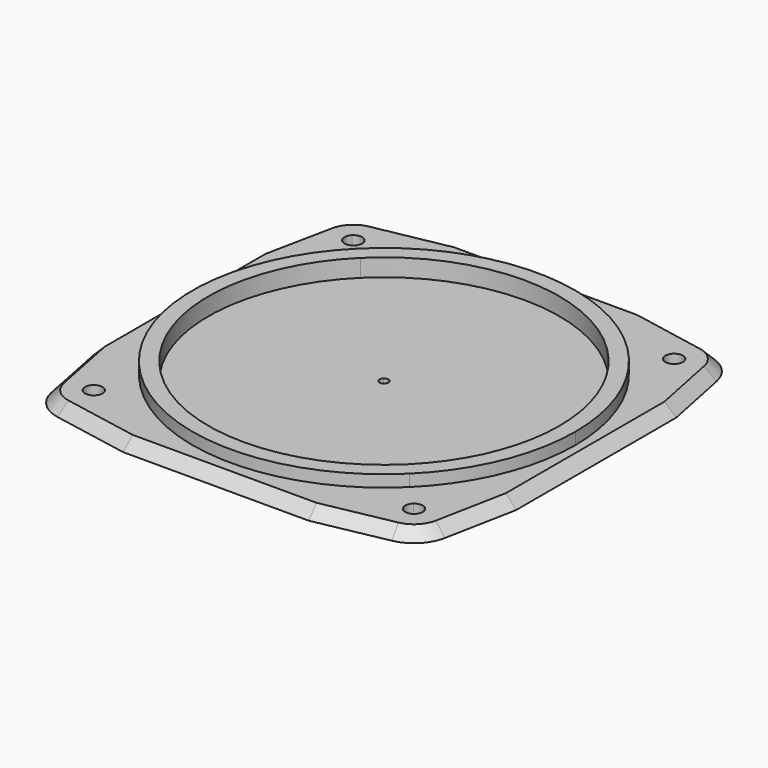
from build123d import *

# Parameters (mm, degrees)
F1_DEPTH     = 0.762
F2_DEPTH     = 3.302
F3_DEPTH     = 1.5875
F4_T1_DEPTH  = 68.7698589568
F4_T3_DEPTH  = 29.8890950425
F4_T5_DEPTH  = 30.9975051116
F4_T7_DEPTH  = 66.2764134385
F4_T9_DEPTH  = 29.6095967996
F4_T11_DEPTH = 30.7124717043
F4_T13_DEPTH = 66.1433332478
F4_T15_DEPTH = 30.7409380137
F4_T17_DEPTH = 29.6692094887
F4_T19_DEPTH = 68.3706865963
F4_T21_DEPTH = 30.237608237
F4_T23_DEPTH = 30.2773753002
F4_T26_ANGLE = 67.887600788
F4_T28_ANGLE = 67.7694142572
F4_T30_ANGLE = 67.6911456036
F4_T32_ANGLE = 68.1706761996


# Not quite as in the source:
# - a fillet or chamfer that OpenCascade refuses, or shapes differently, is made with other operations: its cross-section is extruded or revolved along the edge and cut away or added


with BuildPart() as f1:
    # F0 (on Top) → F1 (new body)
    with BuildSketch(Plane.XY):
        with BuildLine():
            Line((0.4463481019, 0.4516617893), (17.8539240764, 18.0664715723))
            ThreePointArc((17.8539240764, 18.0664715723), (0, 25.4), (-17.8539240764, 18.0664715723))
            Line((-17.8539240764, 18.0664715723), (-0.4463481019, 0.4516617893))
            ThreePointArc((-0.4463481019, 0.4516617893), (0, 0.635), (0.4463481019, 0.4516617893))
        make_face()
        with BuildLine():
            Line((-0.4463481019, 0.4516617893), (-17.8539240764, 18.0664715723))
            ThreePointArc((-17.8539240764, 18.0664715723), (-25.4, 0), (-17.8539240764, -18.0664715723))
            Line((-17.8539240764, -18.0664715723), (-0.4463481019, -0.4516617893))
            ThreePointArc((-0.4463481019, -0.4516617893), (-0.635, 0), (-0.4463481019, 0.4516617893))
        make_face()
        with BuildLine():
            ThreePointArc((-17.8539240764, -18.0664715723), (0, -25.4), (17.8539240764, -18.0664715723))
            Line((17.8539240764, -18.0664715723), (0.4463481019, -0.4516617893))
            ThreePointArc((0.4463481019, -0.4516617893), (0, -0.635), (-0.4463481019, -0.4516617893))
            Line((-0.4463481019, -0.4516617893), (-17.8539240764, -18.0664715723))
        make_face()
        with BuildLine():
            ThreePointArc((17.8539240764, -18.0664715723), (23.4376798291, -9.789543617), (25.4, 0))
            ThreePointArc((25.4, 0), (23.4376798291, 9.789543617), (17.8539240764, 18.0664715723))
            Line((17.8539240764, 18.0664715723), (0.4463481019, 0.4516617893))
            ThreePointArc((0.4463481019, 0.4516617893), (0.5859419957, 0.2447385904), (0.635, 0))
            ThreePointArc((0.635, 0), (0.5859419957, -0.2447385904), (0.4463481019, -0.4516617893))
            Line((0.4463481019, -0.4516617893), (17.8539240764, -18.0664715723))
        make_face()
    extrude(amount=F1_DEPTH)

    # F0 (on Top) → F2 (join)
    with BuildSketch(Plane.XY):
        with BuildLine():
            ThreePointArc((-17.8539240764, 18.0664715723), (0, 25.4), (17.8539240764, 18.0664715723))
            Line((17.8539240764, 18.0664715723), (19.4706182402, 19.7024121658))
            ThreePointArc((19.4706182402, 19.7024121658), (0, 27.7000003576), (-19.4706182402, 19.7024121658))
            Line((-19.4706182402, 19.7024121658), (-17.8539240764, 18.0664715723))
        make_face()
        with BuildLine():
            ThreePointArc((-17.8539240764, -18.0664715723), (-25.4, 0), (-17.8539240764, 18.0664715723))
            Line((-17.8539240764, 18.0664715723), (-19.4706182402, 19.7024121658))
            ThreePointArc((-19.4706182402, 19.7024121658), (-27.7000003576, 0), (-19.4706182402, -19.7024121658))
            Line((-19.4706182402, -19.7024121658), (-17.8539240764, -18.0664715723))
        make_face()
        with BuildLine():
            Line((19.4706182402, -19.7024121658), (17.8539240764, -18.0664715723))
            ThreePointArc((17.8539240764, -18.0664715723), (0, -25.4), (-17.8539240764, -18.0664715723))
            Line((-17.8539240764, -18.0664715723), (-19.4706182402, -19.7024121658))
            ThreePointArc((-19.4706182402, -19.7024121658), (0, -27.7000003576), (19.4706182402, -19.7024121658))
        make_face()
        with BuildLine():
            ThreePointArc((17.8539240764, 18.0664715723), (23.4376798291, 9.789543617), (25.4, 0))
            ThreePointArc((25.4, 0), (23.4376798291, -9.789543617), (17.8539240764, -18.0664715723))
            Line((17.8539240764, -18.0664715723), (19.4706182402, -19.7024121658))
            ThreePointArc((19.4706182402, -19.7024121658), (25.5599897498, -10.6759984918), (27.7000003576, 0))
            ThreePointArc((27.7000003576, 0), (25.5599897498, 10.6759984918), (19.4706182402, 19.7024121658))
            Line((19.4706182402, 19.7024121658), (17.8539240764, 18.0664715723))
        make_face()
    extrude(amount=F2_DEPTH)

    # F0 (on Top) → F3 (join)
    with BuildSketch(Plane.XY):
        with BuildLine():
            ThreePointArc((-19.4706182402, 19.7024121658), (0, 27.7000003576), (19.4706182402, 19.7024121658))
            Line((19.4706182402, 19.7024121658), (22.3259415659, 22.5917275607))
            ThreePointArc((22.3259415659, 22.5917275607), (22.3153141911, 24.3877473432), (24.1113339735, 24.398374718))
            Line((24.1113339735, 24.398374718), (26.7918864226, 27.1108386229))
            Line((26.7918864226, 27.1108386229), (27.6821187888, 28.0116690324))
            ThreePointArc((27.6821187888, 28.0116690324), (26.1722118102, 29.1163410613), (24.4059253481, 29.7330675073))
            Line((24.4059253481, 29.7330675073), (13.4577511535, 31.8168438971))
            Line((13.4577511535, 31.8168438971), (-13.4931333577, 31.8168438971))
            Line((-13.4931333577, 31.8168438971), (-24.4124478948, 29.7336912681))
            ThreePointArc((-24.4124478948, 29.7336912681), (-26.1764044214, 29.1172901956), (-27.6845826781, 28.0141622538))
            Line((-27.6845826781, 28.0141622538), (-26.7918864226, 27.1108386229))
            Line((-26.7918864226, 27.1108386229), (-24.1137970362, 24.4008671029))
            ThreePointArc((-24.1137970362, 24.4008671029), (-22.7321077122, 24.6676976509), (-21.952476244, 23.4961863607))
            ThreePointArc((-21.952476244, 23.4961863607), (-22.0502202295, 23.007600814), (-22.328406695, 22.5942220368))
            Line((-22.328406695, 22.5942220368), (-19.4706182402, 19.7024121658))
        make_face()
        with BuildLine():
            ThreePointArc((-19.4706182402, -19.7024121658), (-27.7000003576, 0), (-19.4706182402, 19.7024121658))
            Line((-19.4706182402, 19.7024121658), (-22.328406695, 22.5942220368))
            ThreePointArc((-22.328406695, 22.5942220368), (-24.1257998226, 22.6034901569), (-24.1137970362, 24.4008671029))
            Line((-24.1137970362, 24.4008671029), (-26.7918864226, 27.1108386229))
            Line((-26.7918864226, 27.1108386229), (-27.6845826781, 28.0141622538))
            ThreePointArc((-27.6845826781, 28.0141622538), (-28.806546627, 26.5195384668), (-29.4448227731, 24.7630342884))
            Line((-29.4448227731, 24.7630342884), (-31.4425267279, 14.9509597699))
            Line((-31.4425267279, 14.9509597699), (-31.4425267279, -14.6264504503))
            Line((-31.4425267279, -14.6264504503), (-29.4338375739, -24.7214172456))
            ThreePointArc((-29.4338375739, -24.7214172456), (-28.7971534061, -26.4922974633), (-27.669411804, -27.9988107734))
            Line((-27.669411804, -27.9988107734), (-26.7918864226, -27.1108386229))
            Line((-26.7918864226, -27.1108386229), (-24.0986269887, -24.385516459))
            ThreePointArc((-24.0986269887, -24.385516459), (-24.1092543635, -22.5894966765), (-22.3132345811, -22.5788693018))
            Line((-22.3132345811, -22.5788693018), (-19.4706182402, -19.7024121658))
        make_face()
        with BuildLine():
            Line((22.3230898006, -22.5888418457), (19.4706182402, -19.7024121658))
            ThreePointArc((19.4706182402, -19.7024121658), (0, -27.7000003576), (-19.4706182402, -19.7024121658))
            Line((-19.4706182402, -19.7024121658), (-22.3132345811, -22.5788693018))
            ThreePointArc((-22.3132345811, -22.5788693018), (-22.0340467935, -22.9927156995), (-21.9359307849, -23.4821928804))
            ThreePointArc((-21.9359307849, -23.4821928804), (-22.7164536041, -24.6540768718), (-24.0986269887, -24.385516459))
            Line((-24.0986269887, -24.385516459), (-26.7918864226, -27.1108386229))
            Line((-26.7918864226, -27.1108386229), (-27.669411804, -27.9988107734))
            ThreePointArc((-27.669411804, -27.9988107734), (-26.1496583495, -29.1086454062), (-24.3713676477, -29.724328486))
            Line((-24.3713676477, -29.724328486), (-13.163754974, -31.8168438971))
            Line((-13.163754974, -31.8168438971), (13.9202097279, -31.8168438971))
            Line((13.9202097279, -31.8168438971), (24.4012740355, -29.7591081974))
            ThreePointArc((24.4012740355, -29.7591081974), (26.1707747188, -29.1285461533), (27.6783635387, -28.0078690768))
            Line((27.6783635387, -28.0078690768), (26.7918864226, -27.1108386229))
            Line((26.7918864226, -27.1108386229), (24.1069762986, -24.3939651657))
            ThreePointArc((24.1069762986, -24.3939651657), (22.2746158391, -24.4207569441), (22.3230898006, -22.5888418457))
        make_face()
        with BuildLine():
            Line((22.3259415659, 22.5917275607), (19.4706182402, 19.7024121658))
            ThreePointArc((19.4706182402, 19.7024121658), (25.5599897498, 10.6759984918), (27.7000003576, 0))
            ThreePointArc((27.7000003576, 0), (25.5599897498, -10.6759984918), (19.4706182402, -19.7024121658))
            Line((19.4706182402, -19.7024121658), (22.3230898006, -22.5888418457))
            ThreePointArc((22.3230898006, -22.5888418457), (23.6913792809, -22.3664758287), (24.4479394177, -23.5280607403))
            ThreePointArc((24.4479394177, -23.5280607403), (24.3596282174, -23.9933687895), (24.1069762986, -24.3939651657))
            Line((24.1069762986, -24.3939651657), (26.7918864226, -27.1108386229))
            Line((26.7918864226, -27.1108386229), (27.6783635387, -28.0078690768))
            ThreePointArc((27.6783635387, -28.0078690768), (28.7879487003, -26.5030054203), (29.411169277, -24.7402263734))
            Line((29.411169277, -24.7402263734), (31.4425267279, -14.2945268971))
            Line((31.4425267279, -14.2945268971), (31.4425267279, 14.8837109626))
            Line((31.4425267279, 14.8837109626), (29.4421670292, 24.7560759433))
            ThreePointArc((29.4421670292, 24.7560759433), (28.8045816259, 26.5149404148), (27.6821187888, 28.0116690324))
            Line((27.6821187888, 28.0116690324), (26.7918864226, 27.1108386229))
            Line((26.7918864226, 27.1108386229), (24.1113339735, 24.398374718))
            ThreePointArc((24.1113339735, 24.398374718), (24.3905217612, 23.9845283202), (24.4886377697, 23.4950511393))
            ThreePointArc((24.4886377697, 23.4950511393), (23.7081149506, 22.3231671479), (22.3259415659, 22.5917275607))
        make_face()
    extrude(amount=F3_DEPTH)

    # F4: chamfer of 2.54 on 12 edges, made by hand

    # F4_s2 → F4_t1 (cut)
    with BuildSketch(Plane.XZ.offset(-34.5471841382)):
        Polygon((-28.9025267279, 1.5875), (-31.4425267279, -0.9525), (-31.4425267279, 1.5875), align=None)
    extrude(amount=F4_T1_DEPTH, mode=Mode.SUBTRACT)

    # F4_s4 → F4_t3 (cut)
    with BuildSketch(Plane(origin=(-2.2222353061, 11.168174818, 0), x_dir=(0, 0, 1), z_dir=(0.1951534433, -0.9807727227, 0))):
        Polygon((1.5875, 31.1523747161), (-0.9525, 33.6923747161), (1.5875, 33.6923747161), align=None)
    extrude(amount=F4_T3_DEPTH, mode=Mode.SUBTRACT)

    # F4_s6 → F4_t5 (cut)
    with BuildSketch(Plane(origin=(-18.1876927678, 3.3957300736, 0), x_dir=(0, 0, 1), z_dir=(0.9830134812, -0.1835333642, 0))):
        Polygon((1.5875, 31.1523747161), (-0.9525, 33.6923747161), (1.5875, 33.6923747161), align=None)
    extrude(amount=F4_T5_DEPTH, mode=Mode.SUBTRACT)

    # F4_s8 → F4_t7 (cut)
    with BuildSketch(Plane.YZ.offset(-32.7599793423)):
        Polygon((-29.2768438971, 1.5875), (-31.8168438971, -0.9525), (-31.8168438971, 1.5875), align=None)
    extrude(amount=F4_T7_DEPTH, mode=Mode.SUBTRACT)

    # F4_s10 → F4_t9 (cut)
    with BuildSketch(Plane(origin=(3.6690463267, 18.0211666908, 0), x_dir=(0, 0, 1), z_dir=(-0.1995036107, -0.9798970912, 0))):
        Polygon((1.5875, 31.2532109374), (-0.9525, 33.7932109374), (1.5875, 33.7932109374), align=None)
    extrude(amount=F4_T9_DEPTH, mode=Mode.SUBTRACT)

    # F4_s12 → F4_t11 (cut)
    with BuildSketch(Plane(origin=(12.0865328675, 2.3058308864, 0), x_dir=(0, 0, 1), z_dir=(-0.9822842374, -0.1873971104, 0))):
        Polygon((1.5875, 31.2417584447), (-0.9525, 33.7817584447), (1.5875, 33.7817584447), align=None)
    extrude(amount=F4_T11_DEPTH, mode=Mode.SUBTRACT)

    # F4_s14 → F4_t13 (cut)
    with BuildSketch(Plane.YZ.offset(-33.089357726)):
        Polygon((29.2768438971, 1.5875), (31.8168438971, -0.9525), (31.8168438971, 1.5875), align=None)
    extrude(amount=F4_T13_DEPTH, mode=Mode.SUBTRACT)

    # F4_s16 → F4_t15 (cut)
    with BuildSketch(Plane(origin=(18.0914247696, -3.4433580544, 0), x_dir=(0, 0, 1), z_dir=(-0.9823647823, 0.1869744218, 0))):
        Polygon((1.5875, 31.2320021705), (-0.9525, 33.7720021705), (1.5875, 33.7720021705), align=None)
    extrude(amount=F4_T15_DEPTH, mode=Mode.SUBTRACT)

    # F4_s18 → F4_t17 (cut)
    with BuildSketch(Plane(origin=(2.2346970165, -11.0288887457, 0), x_dir=(0, 0, 1), z_dir=(-0.1985865833, 0.980083348, 0))):
        Polygon((1.5875, 31.2320021705), (-0.9525, 33.7720021705), (1.5875, 33.7720021705), align=None)
    extrude(amount=F4_T17_DEPTH, mode=Mode.SUBTRACT)

    # F4_s20 → F4_t19 (cut)
    with BuildSketch(Plane.XZ.offset(-34.4799353309)):
        Polygon((28.9025267279, 1.5875), (31.4425267279, -0.9525), (31.4425267279, 1.5875), align=None)
    extrude(amount=F4_T19_DEPTH, mode=Mode.SUBTRACT)

    # F4_s22 → F4_t21 (cut)
    with BuildSketch(Plane(origin=(-3.5641324861, -18.3275753981, 0), x_dir=(0, 0, 1), z_dir=(0.1908922257, 0.9816110015, 0))):
        Polygon((1.5875, 31.053044204), (-0.9525, 33.593044204), (1.5875, 33.593044204), align=None)
    extrude(amount=F4_T21_DEPTH, mode=Mode.SUBTRACT)

    # F4_s24 → F4_t23 (cut)
    with BuildSketch(Plane(origin=(-11.8402934583, -2.3245916472, 0), x_dir=(0, 0, 1), z_dir=(0.9812673161, 0.1926511209, 0))):
        Polygon((1.5875, 31.3625730245), (-0.9525, 33.9025730245), (1.5875, 33.9025730245), align=None)
    extrude(amount=F4_T23_DEPTH, mode=Mode.SUBTRACT)

    # F4_s25 → F4_t26 (revolve, cut)
    with BuildSketch(Plane(origin=(17.8699053405, 3.5083786426, 0), x_dir=(0, 0, 1), z_dir=(-0.9812673161, -0.1926511209, 0))):
        Polygon((1.5875, -31.3625730245), (-0.9525, -33.9025730245), (1.5875, -33.9025730245), align=None)
    revolve(axis=Axis((23.1779394177, -23.5280607403, 1.5875), (0, 0, 1)), revolution_arc=F4_T26_ANGLE, mode=Mode.SUBTRACT)

    # F4_s27 → F4_t28 (revolve, cut)
    with BuildSketch(Plane(origin=(-3.6572099251, 18.0494094211, 0), x_dir=(0, 0, 1), z_dir=(0.1985865833, -0.980083348, 0))):
        Polygon((1.5875, -31.2320021705), (-0.9525, -33.7720021705), (1.5875, -33.7720021705), align=None)
    revolve(axis=Axis((23.2186377697, 23.4950511393, 1.5875), (0, 0, 1)), revolution_arc=F4_T28_ANGLE, mode=Mode.SUBTRACT)

    # F4_s29 → F4_t30 (revolve, cut)
    with BuildSketch(Plane(origin=(-18.081843979, -3.4495975634, 0), x_dir=(0, 0, 1), z_dir=(0.9822842374, 0.1873971104, 0))):
        Polygon((1.5875, -31.2417584447), (-0.9525, -33.7817584447), (1.5875, -33.7817584447), align=None)
    revolve(axis=Axis((-23.222476244, 23.4961863607, 1.5875), (0, 0, 1)), revolution_arc=F4_T30_ANGLE, mode=Mode.SUBTRACT)

    # F4_s31 → F4_t32 (revolve, cut)
    with BuildSketch(Plane(origin=(3.6107245099, -18.1462343053, 0), x_dir=(0, 0, 1), z_dir=(-0.1951534433, 0.9807727227, 0))):
        Polygon((1.5875, -31.1523747161), (-0.9525, -33.6923747161), (1.5875, -33.6923747161), align=None)
    revolve(axis=Axis((-23.2059307849, -23.4821928804, 1.5875), (0, 0, 1)), revolution_arc=F4_T32_ANGLE, mode=Mode.SUBTRACT)


solid = f1.part
